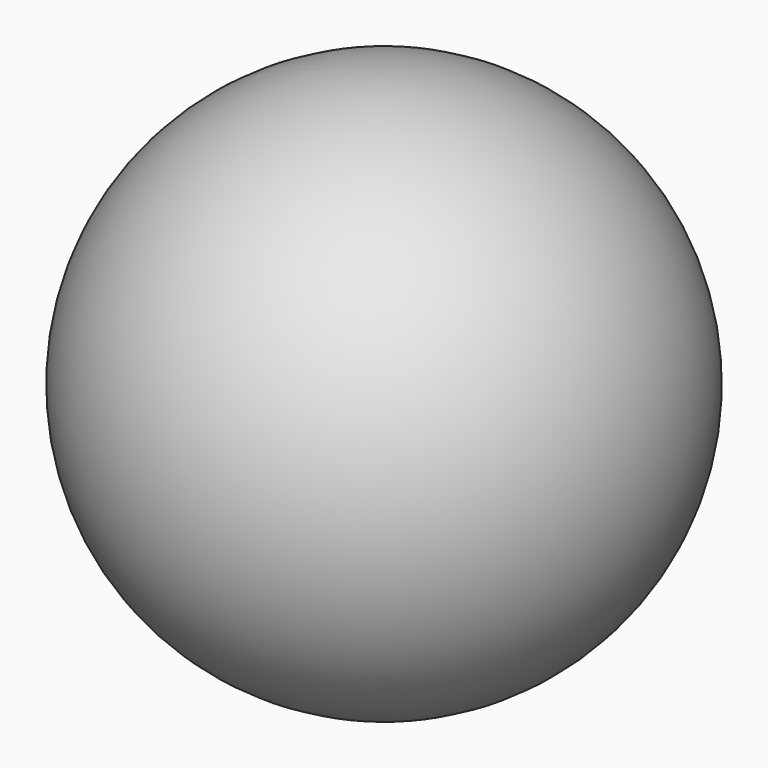
from build123d import *


# Not quite as in the source:
# - the program builds the solid bodies; features that only make, move or delete a surface that nothing else refers to are left out


with BuildPart() as f2:
    # F0 (on Front) → F2 (revolve)
    with BuildSketch(Plane.XZ):
        with BuildLine():
            Line((0, -47.7512898566), (0, 47.7512898566))
            ThreePointArc((0, 47.7512898566), (-47.7512898566, 0), (0, -47.7512898566))
        make_face()
    revolve(axis=Axis((0, 0, 0), (0, 0, 1)))


solid = f2.part
